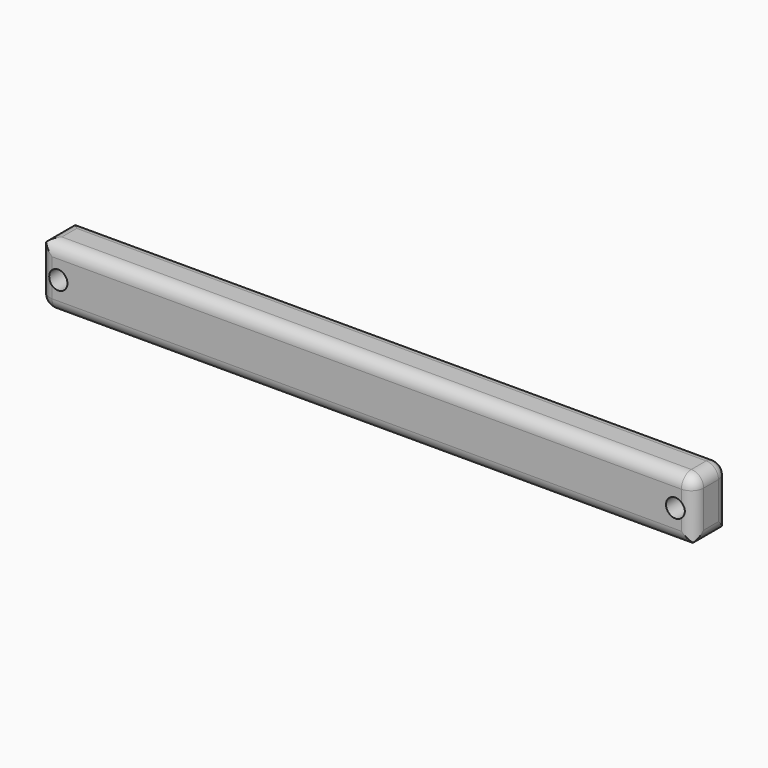
from build123d import *

# Parameters (mm, degrees)
F0_W         = 106
F0_H         = 10
F0_R         = 1.5
F1_DEPTH     = 7
F2_T1_DEPTH  = 17
F2_T3_DEPTH  = 3
F2_T5_DEPTH  = 13
F2_T7_DEPTH  = 109
F2_S11_W     = 2
F2_S11_H     = 2
F2_T12_DEPTH = 2
F2_S17_W     = 2
F2_S17_H     = 2
F2_T18_DEPTH = 2
F3_T1_DEPTH  = 11
F3_T3_DEPTH  = 3
F3_T5_DEPTH  = 107
F3_S9_W      = 2.04
F3_S9_H      = 2.04
F3_T10_DEPTH = 2.04
F3_S15_W     = 2.04
F3_S15_H     = 2.04
F3_T16_DEPTH = 2.04


# Not quite as in the source:
# - a fillet or chamfer that OpenCascade refuses, or shapes differently, is made with other operations: its cross-section is extruded or revolved along the edge and cut away or added


with BuildPart() as f1:
    # F0 (on Front) → F1 (new body)
    with BuildSketch(Plane.XZ):
        with Locations((0, 5)):
            Rectangle(F0_W, F0_H)
        with Locations((-50, 5)):
            Circle(F0_R, mode=Mode.SUBTRACT)
        with Locations((50, 5)):
            Circle(F0_R, mode=Mode.SUBTRACT)
    extrude(amount=F1_DEPTH)

    # F2: fillet of radius 2 on 7 edges, made by hand

    # F2_s2 → F2_t1 (cut)
    with BuildSketch(Plane.XZ.offset(-5)):
        with BuildLine():
            ThreePointArc((51, 0), (52.4142135624, 0.5857864376), (53, 2))
            Line((53, 2), (53, 0))
            Line((53, 0), (51, 0))
        make_face()
        with BuildLine():
            ThreePointArc((-53, 8), (-52.4142135624, 9.4142135624), (-51, 10))
            Line((-51, 10), (-53, 10))
            Line((-53, 10), (-53, 8))
        make_face()
    extrude(amount=F2_T1_DEPTH, mode=Mode.SUBTRACT)

    # F2_s4 → F2_t3 (cut)
    with BuildSketch(Plane.XZ.offset(2)):
        with BuildLine():
            ThreePointArc((53, 8), (52.4142135624, 9.4142135624), (51, 10))
            Line((51, 10), (53, 10))
            Line((53, 10), (53, 8))
        make_face()
    extrude(amount=F2_T3_DEPTH, mode=Mode.SUBTRACT)

    # F2_s6 → F2_t5 (cut)
    with BuildSketch(Plane.XY.offset(-5)):
        with BuildLine():
            ThreePointArc((53, -2), (52.4142135624, -0.5857864376), (51, 0))
            Line((51, 0), (53, 0))
            Line((53, 0), (53, -2))
        make_face()
        with BuildLine():
            ThreePointArc((53, -5), (52.4142135624, -6.4142135624), (51, -7))
            Line((51, -7), (53, -7))
            Line((53, -7), (53, -5))
        make_face()
    extrude(amount=F2_T5_DEPTH, mode=Mode.SUBTRACT)

    # F2_s8 → F2_t7 (cut)
    with BuildSketch(Plane.YZ.offset(-58)):
        with BuildLine():
            ThreePointArc((-2, 10), (-0.5857864376, 9.4142135624), (0, 8))
            Line((0, 8), (0, 10))
            Line((0, 10), (-2, 10))
        make_face()
        with BuildLine():
            ThreePointArc((-5, 10), (-6.4142135624, 9.4142135624), (-7, 8))
            Line((-7, 8), (-7, 10))
            Line((-7, 10), (-5, 10))
        make_face()
    extrude(amount=F2_T7_DEPTH, mode=Mode.SUBTRACT)


with BuildPart() as f2_tool10:
    # F2_s11 → F2_t12 (new body)
    with BuildSketch(Plane.YZ.offset(51)):
        with Locations((-1, 9)):
            Rectangle(F2_S11_W, F2_S11_H)
    extrude(amount=F2_T12_DEPTH)

    # F2_s13 → F2_t14 (revolve, cut)
    with BuildSketch(Plane(origin=(51, -2, 8), x_dir=(0, -0.7071067812, -0.7071067812), z_dir=(0, -0.7071067812, 0.7071067812))):
        with BuildLine():
            ThreePointArc((0, -2), (2, 0), (0, 2))
            Line((0, 2), (0, -2))
        make_face()
    revolve(axis=Axis((51, -2, 8), (1, 0, 0)), mode=Mode.SUBTRACT)


with BuildPart() as f1_1:
    add(f1.part)

    # F2_t9: cut F2_tool10
    add(f2_tool10.part, mode=Mode.SUBTRACT)


with BuildPart() as f2_tool16:
    # F2_s17 → F2_t18 (new body)
    with BuildSketch(Plane.YZ.offset(51)):
        with Locations((-6, 9)):
            Rectangle(F2_S17_W, F2_S17_H)
    extrude(amount=F2_T18_DEPTH)

    # F2_s19 → F2_t20 (revolve, cut)
    with BuildSketch(Plane(origin=(51, -5, 8), x_dir=(0, 0.7071067812, -0.7071067812), z_dir=(0, -0.7071067812, -0.7071067812))):
        with BuildLine():
            ThreePointArc((0, -2), (2, 0), (0, 2))
            Line((0, 2), (0, -2))
        make_face()
    revolve(axis=Axis((51, -5, 8), (1, 0, 0)), mode=Mode.SUBTRACT)


with BuildPart() as f1_2:
    add(f1_1.part)

    # F2_t15: cut F2_tool16
    add(f2_tool16.part, mode=Mode.SUBTRACT)

    # F3: fillet of radius 2 on 7 edges, made by hand

    # F3_s2 → F3_t1 (cut)
    with BuildSketch(Plane.XY.offset(2)):
        with BuildLine():
            ThreePointArc((-53, -2), (-52.4142135624, -0.5857864376), (-51, 0))
            Line((-51, 0), (-53, 0))
            Line((-53, 0), (-53, -2))
        make_face()
        with BuildLine():
            ThreePointArc((-53, -5), (-52.4142135624, -6.4142135624), (-51, -7))
            Line((-51, -7), (-53, -7))
            Line((-53, -7), (-53, -5))
        make_face()
    extrude(amount=F3_T1_DEPTH, mode=Mode.SUBTRACT)

    # F3_s4 → F3_t3 (cut)
    with BuildSketch(Plane.XZ.offset(2)):
        with BuildLine():
            ThreePointArc((-53, 2), (-52.4142135624, 0.5857864376), (-51, 0))
            Line((-51, 0), (-53, 0))
            Line((-53, 0), (-53, 2))
        make_face()
    extrude(amount=F3_T3_DEPTH, mode=Mode.SUBTRACT)

    # F3_s6 → F3_t5 (cut)
    with BuildSketch(Plane.YZ.offset(-51)):
        with BuildLine():
            ThreePointArc((0, 2), (-0.5857864376, 0.5857864376), (-2, 0))
            Line((-2, 0), (0, 0))
            Line((0, 0), (0, 2))
        make_face()
        with BuildLine():
            ThreePointArc((-5, 0), (-6.4142135624, 0.5857864376), (-7, 2))
            Line((-7, 2), (-7, 0))
            Line((-7, 0), (-5, 0))
        make_face()
    extrude(amount=F3_T5_DEPTH, mode=Mode.SUBTRACT)


with BuildPart() as f3_tool8:
    # F3_s9 → F3_t10 (new body)
    with BuildSketch(Plane.YZ.offset(-51)):
        with Locations((-0.98, 0.98)):
            Rectangle(F3_S9_W, F3_S9_H)
    extrude(amount=-F3_T10_DEPTH)

    # F3_s11 → F3_t12 (revolve, cut)
    with BuildSketch(Plane(origin=(-51, -2, 2), x_dir=(0, -0.7071067812, 0.7071067812), z_dir=(0, -0.7071067812, -0.7071067812))):
        with BuildLine():
            ThreePointArc((0, -2), (2, 0), (0, 2))
            Line((0, 2), (0, -2))
        make_face()
    revolve(axis=Axis((-51, -2, 2), (-1, 0, 0)), mode=Mode.SUBTRACT)


with BuildPart() as f1_3:
    add(f1_2.part)

    # F3_t7: cut F3_tool8
    add(f3_tool8.part, mode=Mode.SUBTRACT)


with BuildPart() as f3_tool14:
    # F3_s15 → F3_t16 (new body)
    with BuildSketch(Plane.YZ.offset(-51)):
        with Locations((-6.02, 0.98)):
            Rectangle(F3_S15_W, F3_S15_H)
    extrude(amount=-F3_T16_DEPTH)

    # F3_s17 → F3_t18 (revolve, cut)
    with BuildSketch(Plane(origin=(-51, -5, 2), x_dir=(0, 0.7071067812, 0.7071067812), z_dir=(0, -0.7071067812, 0.7071067812))):
        with BuildLine():
            ThreePointArc((0, -2), (2, 0), (0, 2))
            Line((0, 2), (0, -2))
        make_face()
    revolve(axis=Axis((-51, -5, 2), (-1, 0, 0)), mode=Mode.SUBTRACT)


with BuildPart() as f1_4:
    add(f1_3.part)

    # F3_t13: cut F3_tool14
    add(f3_tool14.part, mode=Mode.SUBTRACT)


solid = f1_4.part
